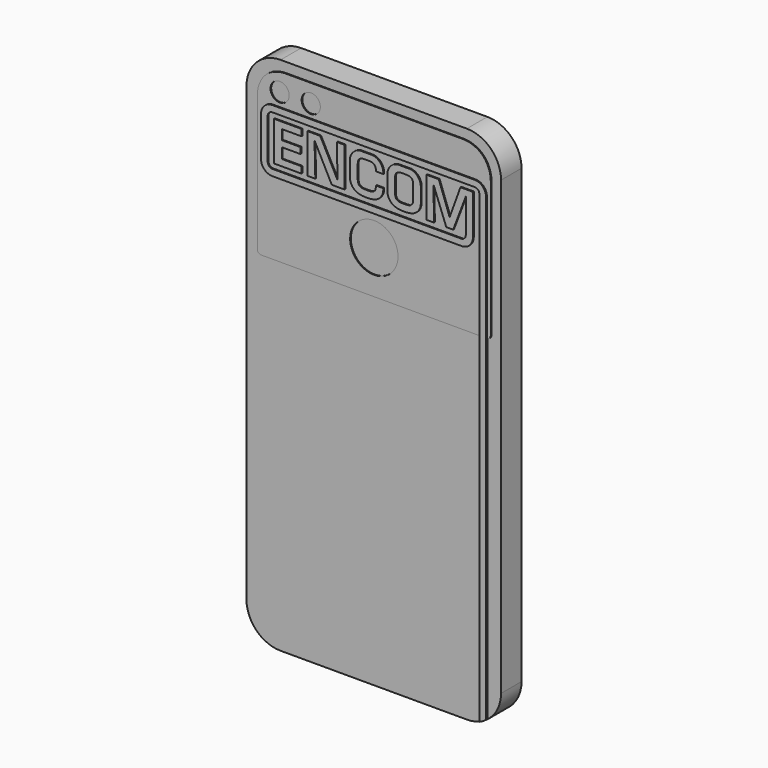
from build123d import *

# Parameters (mm, degrees)
F0_W     = 33.5805061566
F0_H     = 21.1181491613
F0_R     = 2.7798200703
F1_DEPTH = 7.62
F2_DEPTH = 0.254
F3_W     = 56.1288154928
F3_H     = 1.9038211044
F3_W_2   = 1.9916594028
F3_H_2   = 12.0399824588
F3_W_3   = 60.1634240953
F3_H_3   = 1.8881708384
F3_W_4   = 1.9932091236
F3_H_4   = 21.9200883571
F4_DEPTH = 0.5588


with BuildPart() as f1:
    # F0 (on Front) → F1 (new body)
    with BuildSketch(Plane.XZ):
        with BuildLine():
            Line((229.2512688186, 129.6003680688), (201.261898373, 129.6003680688))
            ThreePointArc((201.261898373, 129.6003680688), (194.0776934762, 126.6245729657), (191.101898373, 119.4403680688))
            Line((191.101898373, 119.4403680688), (191.101898373, -14.9256319312))
            ThreePointArc((191.101898373, -14.9256319312), (194.0776934762, -22.109836828), (201.261898373, -25.0856319312))
            Line((201.261898373, -25.0856319312), (229.2512688186, -25.0856319312))
            Line((229.2512688186, -25.0856319312), (229.2512688186, 76.8102183938))
            Line((229.2512688186, 76.8102183938), (195.670762662, 76.8102183938))
            ThreePointArc((195.670762662, 76.8102183938), (194.8754453058, 77.1396496291), (194.5460140705, 77.9349669853))
            Line((194.5460140705, 77.9349669853), (194.5460140705, 118.3175742626))
            ThreePointArc((194.5460140705, 118.3175742626), (194.9559900402, 120.9651454276), (196.1475163698, 123.3647242188))
            ThreePointArc((196.1475163698, 123.3647242188), (197.3925900387, 124.7286537572), (198.9371180534, 125.7410496473))
            ThreePointArc((198.9371180534, 125.7410496473), (200.6644568507, 126.3825901352), (202.4843841791, 126.6709268093))
            Line((202.4843841791, 126.6709268093), (229.2512688186, 126.6709268093))
            Line((229.2512688186, 126.6709268093), (229.2512688186, 129.6003680688))
        make_face()
        with BuildLine():
            Line((256.633898373, 129.6003680688), (229.2512688186, 129.6003680688))
            Line((229.2512688186, 129.6003680688), (229.2512688186, 126.6709268093))
            Line((229.2512688186, 126.6709268093), (256.018153458, 126.6709268093))
            ThreePointArc((256.018153458, 126.6709268093), (257.8380807864, 126.3825901352), (259.5654195837, 125.7410496473))
            ThreePointArc((259.5654195837, 125.7410496473), (261.1099475984, 124.7286537572), (262.3550212673, 123.3647242188))
            ThreePointArc((262.3550212673, 123.3647242188), (263.546547597, 120.9651454276), (263.9565235666, 118.3175742626))
            Line((263.9565235666, 118.3175742626), (263.9565235666, 77.9349669853))
            ThreePointArc((263.9565235666, 77.9349669853), (263.6270923313, 77.1396496291), (262.8317749751, 76.8102183938))
            Line((262.8317749751, 76.8102183938), (229.2512688186, 76.8102183938))
            Line((229.2512688186, 76.8102183938), (229.2512688186, -25.0856319312))
            Line((229.2512688186, -25.0856319312), (256.633898373, -25.0856319312))
            ThreePointArc((256.633898373, -25.0856319312), (263.8181032699, -22.109836828), (266.793898373, -14.9256319312))
            Line((266.793898373, -14.9256319312), (266.793898373, 119.4403680688))
            ThreePointArc((266.793898373, 119.4403680688), (263.8181032699, 126.6245729657), (256.633898373, 129.6003680688))
        make_face()
        with Locations((212.4610157403, 107.7584996819)):
            Rectangle(F0_W, F0_H)
        with Locations((246.0415218969, 107.7584996819)):
            Rectangle(F0_W, F0_H)
        with BuildLine():
            Line((262.8317749751, 97.1994251013), (229.2512688186, 97.1994251013))
            Line((229.2512688186, 97.1994251013), (229.2512688186, 96.7630286436))
            ThreePointArc((229.2512688186, 96.7630286436), (234.2846818006, 94.6781207214), (236.3695897228, 89.6447077394))
            ThreePointArc((236.3695897228, 89.6447077394), (234.2846818006, 84.6112947573), (229.2512688186, 82.5263868351))
            Line((229.2512688186, 82.5263868351), (229.2512688186, 77.9349669853))
            Line((229.2512688186, 77.9349669853), (262.8317749751, 77.9349669853))
            Line((262.8317749751, 77.9349669853), (262.8317749751, 97.1994251013))
        make_face()
        with BuildLine():
            Line((229.2512688186, 96.7630286436), (229.2512688186, 97.1994251013))
            Line((229.2512688186, 97.1994251013), (195.670762662, 97.1994251013))
            Line((195.670762662, 97.1994251013), (195.670762662, 77.9349669853))
            Line((195.670762662, 77.9349669853), (229.2512688186, 77.9349669853))
            Line((229.2512688186, 77.9349669853), (229.2512688186, 82.5263868351))
            ThreePointArc((229.2512688186, 82.5263868351), (222.1329479143, 89.6447077394), (229.2512688186, 96.7630286436))
        make_face()
        with BuildLine():
            Line((229.2512688186, 118.3175742626), (229.2512688186, 126.6709268093))
            Line((229.2512688186, 126.6709268093), (202.4843841791, 126.6709268093))
            ThreePointArc((202.4843841791, 126.6709268093), (200.6644568507, 126.3825901352), (198.9371180534, 125.7410496473))
            ThreePointArc((198.9371180534, 125.7410496473), (197.3925900387, 124.7286537572), (196.1475163698, 123.3647242188))
            ThreePointArc((196.1475163698, 123.3647242188), (194.9559900402, 120.9651454276), (194.5460140705, 118.3175742626))
            Line((194.5460140705, 118.3175742626), (194.5460140705, 77.9349669853))
            ThreePointArc((194.5460140705, 77.9349669853), (194.8754453058, 77.1396496291), (195.670762662, 76.8102183938))
            Line((195.670762662, 76.8102183938), (229.2512688186, 76.8102183938))
            Line((229.2512688186, 76.8102183938), (229.2512688186, 77.9349669853))
            Line((229.2512688186, 77.9349669853), (195.670762662, 77.9349669853))
            Line((195.670762662, 77.9349669853), (195.670762662, 97.1994251013))
            Line((195.670762662, 97.1994251013), (195.670762662, 118.3175742626))
            Line((195.670762662, 118.3175742626), (229.2512688186, 118.3175742626))
        make_face()
        with Locations((201.2345939875, 121.2812513113)):
            Circle(F0_R, mode=Mode.SUBTRACT)
        with Locations((210.4916423559, 121.2812513113)):
            Circle(F0_R, mode=Mode.SUBTRACT)
        with BuildLine():
            Line((256.018153458, 126.6709268093), (229.2512688186, 126.6709268093))
            Line((229.2512688186, 126.6709268093), (229.2512688186, 118.3175742626))
            Line((229.2512688186, 118.3175742626), (262.8317749751, 118.3175742626))
            Line((262.8317749751, 118.3175742626), (262.8317749751, 97.1994251013))
            Line((262.8317749751, 97.1994251013), (262.8317749751, 77.9349669853))
            Line((262.8317749751, 77.9349669853), (229.2512688186, 77.9349669853))
            Line((229.2512688186, 77.9349669853), (229.2512688186, 76.8102183938))
            Line((229.2512688186, 76.8102183938), (262.8317749751, 76.8102183938))
            ThreePointArc((262.8317749751, 76.8102183938), (263.6270923313, 77.1396496291), (263.9565235666, 77.9349669853))
            Line((263.9565235666, 77.9349669853), (263.9565235666, 118.3175742626))
            ThreePointArc((263.9565235666, 118.3175742626), (263.546547597, 120.9651454276), (262.3550212673, 123.3647242188))
            ThreePointArc((262.3550212673, 123.3647242188), (261.1099475984, 124.7286537572), (259.5654195837, 125.7410496473))
            ThreePointArc((259.5654195837, 125.7410496473), (257.8380807864, 126.3825901352), (256.018153458, 126.6709268093))
        make_face()
        with BuildLine():
            ThreePointArc((236.3695897228, 89.6447077394), (234.2846818006, 94.6781207214), (229.2512688186, 96.7630286436))
            Line((229.2512688186, 96.7630286436), (229.2512688186, 82.5263868351))
            ThreePointArc((229.2512688186, 82.5263868351), (234.2846818006, 84.6112947573), (236.3695897228, 89.6447077394))
        make_face()
        with BuildLine():
            Line((229.2512688186, 82.5263868351), (229.2512688186, 96.7630286436))
            ThreePointArc((229.2512688186, 96.7630286436), (222.1329479143, 89.6447077394), (229.2512688186, 82.5263868351))
        make_face()
        with Locations((210.4916423559, 121.2812513113)):
            Circle(F0_R)
        with Locations((201.2345939875, 121.2812513113)):
            Circle(F0_R)
    extrude(amount=-F1_DEPTH)


with BuildPart() as f2:
    # F0 (on Front) → F2 (new body)
    with BuildSketch(Plane.XZ):
        with BuildLine():
            Line((256.018153458, 126.6709268093), (229.2512688186, 126.6709268093))
            Line((229.2512688186, 126.6709268093), (229.2512688186, 118.3175742626))
            Line((229.2512688186, 118.3175742626), (262.8317749751, 118.3175742626))
            Line((262.8317749751, 118.3175742626), (262.8317749751, 97.1994251013))
            Line((262.8317749751, 97.1994251013), (262.8317749751, 77.9349669853))
            Line((262.8317749751, 77.9349669853), (229.2512688186, 77.9349669853))
            Line((229.2512688186, 77.9349669853), (229.2512688186, 76.8102183938))
            Line((229.2512688186, 76.8102183938), (262.8317749751, 76.8102183938))
            ThreePointArc((262.8317749751, 76.8102183938), (263.6270923313, 77.1396496291), (263.9565235666, 77.9349669853))
            Line((263.9565235666, 77.9349669853), (263.9565235666, 118.3175742626))
            ThreePointArc((263.9565235666, 118.3175742626), (263.546547597, 120.9651454276), (262.3550212673, 123.3647242188))
            ThreePointArc((262.3550212673, 123.3647242188), (261.1099475984, 124.7286537572), (259.5654195837, 125.7410496473))
            ThreePointArc((259.5654195837, 125.7410496473), (257.8380807864, 126.3825901352), (256.018153458, 126.6709268093))
        make_face()
        with BuildLine():
            Line((229.2512688186, 118.3175742626), (229.2512688186, 126.6709268093))
            Line((229.2512688186, 126.6709268093), (202.4843841791, 126.6709268093))
            ThreePointArc((202.4843841791, 126.6709268093), (200.6644568507, 126.3825901352), (198.9371180534, 125.7410496473))
            ThreePointArc((198.9371180534, 125.7410496473), (197.3925900387, 124.7286537572), (196.1475163698, 123.3647242188))
            ThreePointArc((196.1475163698, 123.3647242188), (194.9559900402, 120.9651454276), (194.5460140705, 118.3175742626))
            Line((194.5460140705, 118.3175742626), (194.5460140705, 77.9349669853))
            ThreePointArc((194.5460140705, 77.9349669853), (194.8754453058, 77.1396496291), (195.670762662, 76.8102183938))
            Line((195.670762662, 76.8102183938), (229.2512688186, 76.8102183938))
            Line((229.2512688186, 76.8102183938), (229.2512688186, 77.9349669853))
            Line((229.2512688186, 77.9349669853), (195.670762662, 77.9349669853))
            Line((195.670762662, 77.9349669853), (195.670762662, 97.1994251013))
            Line((195.670762662, 97.1994251013), (195.670762662, 118.3175742626))
            Line((195.670762662, 118.3175742626), (229.2512688186, 118.3175742626))
        make_face()
        with Locations((201.2345939875, 121.2812513113)):
            Circle(F0_R, mode=Mode.SUBTRACT)
        with Locations((210.4916423559, 121.2812513113)):
            Circle(F0_R, mode=Mode.SUBTRACT)
        with Locations((212.4610157403, 107.7584996819)):
            Rectangle(F0_W, F0_H)
        with BuildLine():
            Line((229.2512688186, 96.7630286436), (229.2512688186, 97.1994251013))
            Line((229.2512688186, 97.1994251013), (195.670762662, 97.1994251013))
            Line((195.670762662, 97.1994251013), (195.670762662, 77.9349669853))
            Line((195.670762662, 77.9349669853), (229.2512688186, 77.9349669853))
            Line((229.2512688186, 77.9349669853), (229.2512688186, 82.5263868351))
            ThreePointArc((229.2512688186, 82.5263868351), (222.1329479143, 89.6447077394), (229.2512688186, 96.7630286436))
        make_face()
        with BuildLine():
            Line((262.8317749751, 97.1994251013), (229.2512688186, 97.1994251013))
            Line((229.2512688186, 97.1994251013), (229.2512688186, 96.7630286436))
            ThreePointArc((229.2512688186, 96.7630286436), (234.2846818006, 94.6781207214), (236.3695897228, 89.6447077394))
            ThreePointArc((236.3695897228, 89.6447077394), (234.2846818006, 84.6112947573), (229.2512688186, 82.5263868351))
            Line((229.2512688186, 82.5263868351), (229.2512688186, 77.9349669853))
            Line((229.2512688186, 77.9349669853), (262.8317749751, 77.9349669853))
            Line((262.8317749751, 77.9349669853), (262.8317749751, 97.1994251013))
        make_face()
        with Locations((246.0415218969, 107.7584996819)):
            Rectangle(F0_W, F0_H)
    extrude(amount=F2_DEPTH)

    # F3 (on Front) → F4 (join)
    with BuildSketch(Plane.XZ):
        Polygon((199.7636705637, 102.2084653378), (207.9194486141, 102.2084653378), (207.9194486141, 104.1282191873), (202.0396590233, 104.1282191873), (202.0396590233, 107.2249636054), (207.5955271721, 107.2249636054), (207.5955271721, 108.1428825855), (207.5955271721, 109.0608015656), (202.0404785872, 109.0608015656), (202.0404785872, 111.972540617), (207.9194486141, 111.972540617), (207.9194486141, 113.9081418514), (199.7636705637, 113.9081418514), align=None)
        Polygon((218.5415214992, 108.1428825855), (220.7203507423, 108.1428825855), (220.7203507423, 113.9081418514), (218.4271961451, 113.9081418514), align=None)
        Polygon((216.9222682714, 102.2084653378), (220.7203507423, 102.2084653378), (220.7203507423, 108.1428825855), (218.5415214992, 108.1428825855), (218.6210900545, 104.1303575039), (218.5589185962, 104.129124641), (216.466729666, 108.1428825855), (213.8594988403, 108.1428825855), align=None)
        Polygon((211.8716859322, 111.9944657598), (213.8594988403, 108.1428825855), (216.466729666, 108.1428825855), (213.4615629911, 113.9081418514), (209.6930146217, 113.9081418514), (209.6930146217, 108.1428825855), (211.8812335809, 108.1428825855), (211.7895185947, 111.992508173), align=None)
        Polygon((209.6930146217, 102.2084653378), (212.0226174593, 102.2084653378), (211.8812335809, 108.1428825855), (209.6930146217, 108.1428825855), align=None)
        with BuildLine():
            Line((237.8193736076, 112.0741516352), (238.4150922298, 112.0741516352))
            Line((238.4150922298, 112.0741516352), (238.4150922298, 113.9081418514))
            Line((238.4150922298, 113.9081418514), (236.5544438362, 113.9081418514))
            ThreePointArc((236.5544438362, 113.9081418514), (236.3760720746, 113.8790212582), (236.1993858825, 113.8409885906))
            ThreePointArc((236.1993858825, 113.8409885906), (234.406717709, 112.7914019816), (233.4919741893, 110.9263187333))
            ThreePointArc((233.4919741893, 110.9263187333), (233.4804676636, 110.8516665608), (233.4705293179, 110.7767894864))
            Line((233.4705293179, 110.7767894864), (233.4260046482, 110.2137640119))
            Line((233.4260046482, 110.2137640119), (233.4260046482, 108.1428825855))
            Line((233.4260046482, 108.1428825855), (235.7074469328, 108.1428825855))
            Line((235.7074469328, 108.1428825855), (235.7074469328, 110.119998455))
            ThreePointArc((235.7074469328, 110.119998455), (235.7176531546, 110.2203330886), (235.7326234029, 110.3200682244))
            ThreePointArc((235.7326234029, 110.3200682244), (235.7389398189, 110.3974798809), (235.748488876, 110.4745595618))
            ThreePointArc((235.748488876, 110.4745595618), (235.7565008871, 110.5798212659), (235.7712805637, 110.684347721))
            ThreePointArc((235.7712805637, 110.684347721), (235.7927284766, 110.8131717547), (235.8253023796, 110.9396414565))
            ThreePointArc((235.8253023796, 110.9396414565), (235.8453327429, 111.0025957281), (235.8681549799, 111.0645925123))
            ThreePointArc((235.8681549799, 111.0645925123), (235.8976925729, 111.1509776233), (235.9335179955, 111.2349502134))
            ThreePointArc((235.9335179955, 111.2349502134), (236.1113058429, 111.5308226696), (236.3807154714, 111.7466176673))
            ThreePointArc((236.3807154714, 111.7466176673), (236.5149337847, 111.82207606), (236.6574833462, 111.8802838529))
            ThreePointArc((236.6574833462, 111.8802838529), (236.7353133018, 111.91133184), (236.8147769734, 111.9379213941))
            ThreePointArc((236.8147769734, 111.9379213941), (237.0337352549, 112.0021574719), (237.2594984469, 112.035323476))
            ThreePointArc((237.2594984469, 112.035323476), (237.4351597426, 112.0580823334), (237.6121905096, 112.0639953609))
            ThreePointArc((237.6121905096, 112.0639953609), (237.7156576662, 112.0716110431), (237.8193736076, 112.0741516352))
        make_face()
        with BuildLine():
            Line((241.1227375269, 108.1428825855), (243.4041798115, 108.1428825855))
            Line((243.4041798115, 108.1428825855), (243.4041798115, 110.2137640119))
            Line((243.4041798115, 110.2137640119), (243.3596551418, 110.7767894864))
            ThreePointArc((243.3596551418, 110.7767894864), (243.3497167961, 110.8516665608), (243.3382102704, 110.9263187333))
            ThreePointArc((243.3382102704, 110.9263187333), (242.4234667507, 112.7914019816), (240.6307985772, 113.8409885906))
            ThreePointArc((240.6307985772, 113.8409885906), (240.4541123851, 113.8790212582), (240.2757406235, 113.9081418514))
            Line((240.2757406235, 113.9081418514), (238.4150922298, 113.9081418514))
            Line((238.4150922298, 113.9081418514), (238.4150922298, 112.0741516352))
            Line((238.4150922298, 112.0741516352), (239.0108108521, 112.0741516352))
            ThreePointArc((239.0108108521, 112.0741516352), (239.1145267935, 112.0716110431), (239.2179939501, 112.0639953609))
            ThreePointArc((239.2179939501, 112.0639953609), (239.3950247171, 112.0580823334), (239.5706860128, 112.035323476))
            ThreePointArc((239.5706860128, 112.035323476), (239.7964492048, 112.0021574719), (240.0154074862, 111.9379213941))
            ThreePointArc((240.0154074862, 111.9379213941), (240.0948711579, 111.91133184), (240.1727011135, 111.8802838529))
            ThreePointArc((240.1727011135, 111.8802838529), (240.315250675, 111.82207606), (240.4494689882, 111.7466176673))
            ThreePointArc((240.4494689882, 111.7466176673), (240.7188786168, 111.5308226696), (240.8966664642, 111.2349502134))
            ThreePointArc((240.8966664642, 111.2349502134), (240.9324918868, 111.1509776233), (240.9620294798, 111.0645925123))
            ThreePointArc((240.9620294798, 111.0645925123), (240.9848517168, 111.0025957281), (241.0048820801, 110.9396414565))
            ThreePointArc((241.0048820801, 110.9396414565), (241.0374559831, 110.8131717547), (241.058903896, 110.684347721))
            ThreePointArc((241.058903896, 110.684347721), (241.0736835726, 110.5798212659), (241.0816955837, 110.4745595618))
            ThreePointArc((241.0816955837, 110.4745595618), (241.0912446408, 110.3974798809), (241.0975610568, 110.3200682244))
            ThreePointArc((241.0975610568, 110.3200682244), (241.1125313051, 110.2203330886), (241.1227375269, 110.119998455))
            Line((241.1227375269, 110.119998455), (241.1227375269, 108.1428825855))
        make_face()
        with BuildLine():
            Line((238.4150922298, 104.2116135359), (238.4150922298, 102.2084653378))
            ThreePointArc((238.4150922298, 102.2084653378), (239.3492531993, 102.2508418573), (240.2757406235, 102.3776233196))
            ThreePointArc((240.2757406235, 102.3776233196), (240.4541123851, 102.4067439128), (240.6307985772, 102.4447765804))
            ThreePointArc((240.6307985772, 102.4447765804), (242.4234667507, 103.4943631894), (243.3382102704, 105.3594464377))
            ThreePointArc((243.3382102704, 105.3594464377), (243.3497167961, 105.4340986102), (243.3596551418, 105.5089756846))
            Line((243.3596551418, 105.5089756846), (243.4041798115, 106.0720011592))
            Line((243.4041798115, 106.0720011592), (243.4041798115, 108.1428825855))
            Line((243.4041798115, 108.1428825855), (241.1227375269, 108.1428825855))
            Line((241.1227375269, 108.1428825855), (241.1227375269, 106.165766716))
            ThreePointArc((241.1227375269, 106.165766716), (241.1125313051, 106.0654320825), (241.0975610568, 105.9656969467))
            ThreePointArc((241.0975610568, 105.9656969467), (241.0912446408, 105.8882852901), (241.0816955837, 105.8112056093))
            ThreePointArc((241.0816955837, 105.8112056093), (241.0736835726, 105.7059439052), (241.058903896, 105.60141745))
            ThreePointArc((241.058903896, 105.60141745), (241.0374559831, 105.4725934163), (241.0048820801, 105.3461237145))
            ThreePointArc((241.0048820801, 105.3461237145), (240.9848517168, 105.283169443), (240.9620294798, 105.2211726587))
            ThreePointArc((240.9620294798, 105.2211726587), (240.9324918868, 105.1347875478), (240.8966664642, 105.0508149576))
            ThreePointArc((240.8966664642, 105.0508149576), (240.7188786168, 104.7549425014), (240.4494689882, 104.5391475037))
            ThreePointArc((240.4494689882, 104.5391475037), (240.315250675, 104.4636891111), (240.1727011135, 104.4054813182))
            ThreePointArc((240.1727011135, 104.4054813182), (240.0948711579, 104.3744333311), (240.0154074862, 104.347843777))
            ThreePointArc((240.0154074862, 104.347843777), (239.7964492048, 104.2836076991), (239.5706860128, 104.250441695))
            ThreePointArc((239.5706860128, 104.250441695), (239.3950247171, 104.2276828377), (239.2179939501, 104.2217698101))
            ThreePointArc((239.2179939501, 104.2217698101), (239.1145267935, 104.214154128), (239.0108108521, 104.2116135359))
            Line((239.0108108521, 104.2116135359), (238.4150922298, 104.2116135359))
        make_face()
        with BuildLine():
            ThreePointArc((236.5544438362, 102.3776233196), (237.4809312604, 102.2508418573), (238.4150922298, 102.2084653378))
            Line((238.4150922298, 102.2084653378), (238.4150922298, 104.2116135359))
            Line((238.4150922298, 104.2116135359), (237.8193736076, 104.2116135359))
            ThreePointArc((237.8193736076, 104.2116135359), (237.7156576662, 104.214154128), (237.6121905096, 104.2217698101))
            ThreePointArc((237.6121905096, 104.2217698101), (237.4351597426, 104.2276828377), (237.2594984469, 104.250441695))
            ThreePointArc((237.2594984469, 104.250441695), (237.0337352549, 104.2836076991), (236.8147769734, 104.347843777))
            ThreePointArc((236.8147769734, 104.347843777), (236.7353133018, 104.3744333311), (236.6574833462, 104.4054813182))
            ThreePointArc((236.6574833462, 104.4054813182), (236.5149337847, 104.4636891111), (236.3807154714, 104.5391475037))
            ThreePointArc((236.3807154714, 104.5391475037), (236.1113058429, 104.7549425014), (235.9335179955, 105.0508149576))
            ThreePointArc((235.9335179955, 105.0508149576), (235.8976925729, 105.1347875478), (235.8681549799, 105.2211726587))
            ThreePointArc((235.8681549799, 105.2211726587), (235.8453327429, 105.283169443), (235.8253023796, 105.3461237145))
            ThreePointArc((235.8253023796, 105.3461237145), (235.7927284766, 105.4725934163), (235.7712805637, 105.60141745))
            ThreePointArc((235.7712805637, 105.60141745), (235.7565008871, 105.7059439052), (235.748488876, 105.8112056093))
            ThreePointArc((235.748488876, 105.8112056093), (235.7389398189, 105.8882852901), (235.7326234029, 105.9656969467))
            ThreePointArc((235.7326234029, 105.9656969467), (235.7176531546, 106.0654320825), (235.7074469328, 106.165766716))
            Line((235.7074469328, 106.165766716), (235.7074469328, 108.1428825855))
            Line((235.7074469328, 108.1428825855), (233.4260046482, 108.1428825855))
            Line((233.4260046482, 108.1428825855), (233.4260046482, 106.0720011592))
            Line((233.4260046482, 106.0720011592), (233.4705293179, 105.5089756846))
            ThreePointArc((233.4705293179, 105.5089756846), (233.4804676636, 105.4340986102), (233.4919741893, 105.3594464377))
            ThreePointArc((233.4919741893, 105.3594464377), (234.406717709, 103.4943631894), (236.1993858825, 102.4447765804))
            ThreePointArc((236.1993858825, 102.4447765804), (236.3760720746, 102.4067439128), (236.5544438362, 102.3776233196))
        make_face()
        with BuildLine():
            Line((227.3379266262, 113.9081418514), (227.3379266262, 112.0741516352))
            Line((227.3379266262, 112.0741516352), (227.3467183113, 112.0741516352))
            Line((227.3467183113, 112.0741516352), (227.9424369335, 112.0741516352))
            ThreePointArc((227.9424369335, 112.0741516352), (228.0461528749, 112.0716110431), (228.1496200316, 112.0639953609))
            ThreePointArc((228.1496200316, 112.0639953609), (228.3266507986, 112.0580823334), (228.5023120942, 112.035323476))
            ThreePointArc((228.5023120942, 112.035323476), (228.7280752863, 112.0021574719), (228.9470335677, 111.9379213941))
            ThreePointArc((228.9470335677, 111.9379213941), (229.0264972393, 111.91133184), (229.104327195, 111.8802838529))
            ThreePointArc((229.104327195, 111.8802838529), (229.2468767565, 111.82207606), (229.3810950697, 111.7466176673))
            ThreePointArc((229.3810950697, 111.7466176673), (229.6505046983, 111.5308226696), (229.8282925456, 111.2349502134))
            ThreePointArc((229.8282925456, 111.2349502134), (229.8641179682, 111.1509776233), (229.8936555612, 111.0645925123))
            ThreePointArc((229.8936555612, 111.0645925123), (229.9164777982, 111.0025957281), (229.9365081615, 110.9396414565))
            ThreePointArc((229.9365081615, 110.9396414565), (229.9690820646, 110.8131717547), (229.9905299775, 110.684347721))
            ThreePointArc((229.9905299775, 110.684347721), (230.0053096541, 110.5798212659), (230.0133216651, 110.4745595618))
            ThreePointArc((230.0133216651, 110.4745595618), (230.0228707222, 110.3974798809), (230.0291871382, 110.3200682244))
            ThreePointArc((230.0291871382, 110.3200682244), (230.0441573866, 110.2203330886), (230.0543636084, 110.119998455))
            Line((230.0543636084, 110.119998455), (230.0543636084, 109.9947020411))
            Line((230.0543636084, 109.9947020411), (232.2537600994, 109.9947020411))
            Line((232.2537600994, 109.9947020411), (232.2537600994, 110.2149261945))
            Line((232.2537600994, 110.2149261945), (232.2092354298, 110.777951669))
            ThreePointArc((232.2092354298, 110.777951669), (232.199297084, 110.8528287434), (232.1877905583, 110.9274809159))
            ThreePointArc((232.1877905583, 110.9274809159), (231.2730470386, 112.7925641643), (229.4803788651, 113.8421507732))
            ThreePointArc((229.4803788651, 113.8421507732), (229.3078455553, 113.8793954681), (229.1336945986, 113.9081418514))
            Line((229.1336945986, 113.9081418514), (227.3379266262, 113.9081418514))
        make_face()
        with BuildLine():
            Line((222.2755849361, 108.1440447681), (222.2755849361, 108.1428825855))
            Line((222.2755849361, 108.1428825855), (224.6214896441, 108.1428825855))
            Line((224.6214896441, 108.1428825855), (224.6214896441, 110.119998455))
            ThreePointArc((224.6214896441, 110.119998455), (224.6316958658, 110.2203330886), (224.6466661142, 110.3200682244))
            ThreePointArc((224.6466661142, 110.3200682244), (224.6529825302, 110.3974798809), (224.6625315873, 110.4745595618))
            ThreePointArc((224.6625315873, 110.4745595618), (224.6705435983, 110.5798212659), (224.6853232749, 110.684347721))
            ThreePointArc((224.6853232749, 110.684347721), (224.7067711878, 110.8131717547), (224.7393450909, 110.9396414565))
            ThreePointArc((224.7393450909, 110.9396414565), (224.7593754542, 111.0025957281), (224.7821976912, 111.0645925123))
            ThreePointArc((224.7821976912, 111.0645925123), (224.8117352842, 111.1509776233), (224.8475607068, 111.2349502134))
            ThreePointArc((224.8475607068, 111.2349502134), (225.0253485541, 111.5308226696), (225.2947581827, 111.7466176673))
            ThreePointArc((225.2947581827, 111.7466176673), (225.428976496, 111.82207606), (225.5715260574, 111.8802838529))
            ThreePointArc((225.5715260574, 111.8802838529), (225.6493560131, 111.91133184), (225.7288196847, 111.9379213941))
            ThreePointArc((225.7288196847, 111.9379213941), (225.9477779661, 112.0021574719), (226.1735411582, 112.035323476))
            ThreePointArc((226.1735411582, 112.035323476), (226.3492024538, 112.0580823334), (226.5262332209, 112.0639953609))
            ThreePointArc((226.5262332209, 112.0639953609), (226.6297003775, 112.0716110431), (226.7334163189, 112.0741516352))
            Line((226.7334163189, 112.0741516352), (227.3291349411, 112.0741516352))
            Line((227.3291349411, 112.0741516352), (227.3379266262, 112.0741516352))
            Line((227.3379266262, 112.0741516352), (227.3379266262, 113.9081418514))
            Line((227.3379266262, 113.9081418514), (225.3956504369, 113.9081418514))
            ThreePointArc((225.3956504369, 113.9081418514), (225.2214994802, 113.8793954681), (225.0489661704, 113.8421507732))
            ThreePointArc((225.0489661704, 113.8421507732), (223.2562979969, 112.7925641643), (222.3415544772, 110.9274809159))
            ThreePointArc((222.3415544772, 110.9274809159), (222.3300479516, 110.8528287434), (222.3201096058, 110.777951669))
            Line((222.3201096058, 110.777951669), (222.2755849361, 110.2149261945))
            Line((222.2755849361, 110.2149261945), (222.2755849361, 108.1440447681))
        make_face()
        with BuildLine():
            ThreePointArc((225.4040241241, 102.3787855022), (226.3669942845, 102.2487525493), (227.3379266262, 102.2098875714))
            Line((227.3379266262, 102.2098875714), (227.3379266262, 104.2116135359))
            Line((227.3379266262, 104.2116135359), (227.3291349411, 104.2116135359))
            Line((227.3291349411, 104.2116135359), (226.7334163189, 104.2116135359))
            ThreePointArc((226.7334163189, 104.2116135359), (226.6297003775, 104.214154128), (226.5262332209, 104.2217698101))
            ThreePointArc((226.5262332209, 104.2217698101), (226.3492024538, 104.2276828377), (226.1735411582, 104.250441695))
            ThreePointArc((226.1735411582, 104.250441695), (225.9477779661, 104.2836076991), (225.7288196847, 104.347843777))
            ThreePointArc((225.7288196847, 104.347843777), (225.6493560131, 104.3744333311), (225.5715260574, 104.4054813182))
            ThreePointArc((225.5715260574, 104.4054813182), (225.428976496, 104.4636891111), (225.2947581827, 104.5391475037))
            ThreePointArc((225.2947581827, 104.5391475037), (225.0253485541, 104.7549425014), (224.8475607068, 105.0508149576))
            ThreePointArc((224.8475607068, 105.0508149576), (224.8117352842, 105.1347875478), (224.7821976912, 105.2211726587))
            ThreePointArc((224.7821976912, 105.2211726587), (224.7593754542, 105.283169443), (224.7393450909, 105.3461237145))
            ThreePointArc((224.7393450909, 105.3461237145), (224.7067711878, 105.4725934163), (224.6853232749, 105.60141745))
            ThreePointArc((224.6853232749, 105.60141745), (224.6705435983, 105.7059439052), (224.6625315873, 105.8112056093))
            ThreePointArc((224.6625315873, 105.8112056093), (224.6529825302, 105.8882852901), (224.6466661142, 105.9656969467))
            ThreePointArc((224.6466661142, 105.9656969467), (224.6316958658, 106.0654320825), (224.6214896441, 106.165766716))
            Line((224.6214896441, 106.165766716), (224.6214896441, 108.1428825855))
            Line((224.6214896441, 108.1428825855), (222.2755849361, 108.1428825855))
            Line((222.2755849361, 108.1428825855), (222.2755849361, 106.0731633418))
            Line((222.2755849361, 106.0731633418), (222.3201096058, 105.5101378673))
            ThreePointArc((222.3201096058, 105.5101378673), (222.3300479516, 105.4352607928), (222.3415544772, 105.3606086204))
            ThreePointArc((222.3415544772, 105.3606086204), (223.2562979969, 103.495525372), (225.0489661704, 102.445938763))
            ThreePointArc((225.0489661704, 102.445938763), (225.2256523625, 102.4079060955), (225.4040241241, 102.3787855022))
        make_face()
        with BuildLine():
            Line((227.3379266262, 104.2116135359), (227.3379266262, 102.2098875714))
            ThreePointArc((227.3379266262, 102.2098875714), (228.2353044509, 102.2553850225), (229.1253209114, 102.3787855022))
            ThreePointArc((229.1253209114, 102.3787855022), (229.303692673, 102.4079060955), (229.4803788651, 102.445938763))
            ThreePointArc((229.4803788651, 102.445938763), (231.2730470386, 103.495525372), (232.1877905583, 105.3606086204))
            ThreePointArc((232.1877905583, 105.3606086204), (232.199297084, 105.4352607928), (232.2092354298, 105.5101378673))
            Line((232.2092354298, 105.5101378673), (232.2537600994, 106.0731633418))
            Line((232.2537600994, 106.0731633418), (232.2537600994, 106.2910631299))
            Line((232.2537600994, 106.2910631299), (230.0543636084, 106.2910631299))
            Line((230.0543636084, 106.2910631299), (230.0543636084, 106.165766716))
            ThreePointArc((230.0543636084, 106.165766716), (230.0441573866, 106.0654320825), (230.0291871382, 105.9656969467))
            ThreePointArc((230.0291871382, 105.9656969467), (230.0228707222, 105.8882852901), (230.0133216651, 105.8112056093))
            ThreePointArc((230.0133216651, 105.8112056093), (230.0053096541, 105.7059439052), (229.9905299775, 105.60141745))
            ThreePointArc((229.9905299775, 105.60141745), (229.9690820646, 105.4725934163), (229.9365081615, 105.3461237145))
            ThreePointArc((229.9365081615, 105.3461237145), (229.9164777982, 105.283169443), (229.8936555612, 105.2211726587))
            ThreePointArc((229.8936555612, 105.2211726587), (229.8641179682, 105.1347875478), (229.8282925456, 105.0508149576))
            ThreePointArc((229.8282925456, 105.0508149576), (229.6505046983, 104.7549425014), (229.3810950697, 104.5391475037))
            ThreePointArc((229.3810950697, 104.5391475037), (229.2468767565, 104.4636891111), (229.104327195, 104.4054813182))
            ThreePointArc((229.104327195, 104.4054813182), (229.0264972393, 104.3744333311), (228.9470335677, 104.347843777))
            ThreePointArc((228.9470335677, 104.347843777), (228.7280752863, 104.2836076991), (228.5023120942, 104.250441695))
            ThreePointArc((228.5023120942, 104.250441695), (228.3266507986, 104.2276828377), (228.1496200316, 104.2217698101))
            ThreePointArc((228.1496200316, 104.2217698101), (228.0461528749, 104.214154128), (227.9424369335, 104.2116135359))
            Line((227.9424369335, 104.2116135359), (227.3467183113, 104.2116135359))
            Line((227.3467183113, 104.2116135359), (227.3379266262, 104.2116135359))
        make_face()
        Polygon((256.7622959614, 102.2084653378), (256.7622959614, 102.0197641448), (258.8952766269, 102.0197641448), (258.902490139, 114.0043064952), (255.1763653755, 114.0043064952), (251.9906163216, 105.2259132266), (251.9319951534, 105.2259132266), (248.7232983112, 114.0043064952), (245.0365126133, 114.0043064952), (245.0365126133, 113.9081418514), (245.0365126133, 108.1428825855), (245.0365126133, 102.2084653378), (247.3303228617, 102.2084653378), (247.1502870321, 112.0081096888), (247.2019113399, 112.0090581135), (250.9705126286, 102.2084653378), (253.0142366886, 102.2084653378), (256.7622959614, 112.0972558856), align=None)
        with BuildLine():
            Line((255.3781572386, 100.635625422), (255.3781572386, 98.7318043176))
            Line((255.3781572386, 98.7318043176), (255.6793465587, 98.7318043176))
            ThreePointArc((255.6793465587, 98.7318043176), (257.9360745098, 99.7412338469), (258.8952766269, 102.0197641448))
            Line((258.8952766269, 102.0197641448), (256.7622959614, 102.0197641448))
            ThreePointArc((256.7622959614, 102.0197641448), (256.3568911156, 101.0410302678), (255.3781572386, 100.635625422))
        make_face()
        with Locations((227.3137494922, 99.6837148698)):
            Rectangle(F3_W, F3_H)
        with Locations((196.8693733215, 108.0397553742)):
            Rectangle(F3_W_2, F3_H_2)
        with BuildLine():
            Line((197.865203023, 102.0197641448), (195.8735436201, 102.0197641448))
            ThreePointArc((195.8735436201, 102.0197641448), (196.8952727919, 99.69181752), (199.2493417458, 98.7318043176))
            Line((199.2493417458, 98.7318043176), (199.2493417458, 100.635625422))
            ThreePointArc((199.2493417458, 100.635625422), (198.2706078688, 101.0410302678), (197.865203023, 102.0197641448))
        make_face()
        with BuildLine():
            Line((199.2493417458, 115.4438853264), (199.2493417458, 117.3320561647))
            ThreePointArc((199.2493417458, 117.3320561647), (196.8921665513, 116.3863437364), (195.8735436201, 114.0597466036))
            Line((195.8735436201, 114.0597466036), (197.865203023, 114.0597466036))
            ThreePointArc((197.865203023, 114.0597466036), (198.2706078688, 115.0384804806), (199.2493417458, 115.4438853264))
        make_face()
        with Locations((229.3310537934, 116.3879707456)):
            Rectangle(F3_W_3, F3_H_3)
        with BuildLine():
            ThreePointArc((262.7901136875, 114.0597466036), (261.7661640256, 116.381962715), (259.4127658411, 117.3320561647))
            Line((259.4127658411, 117.3320561647), (259.4127658411, 115.4438853264))
            ThreePointArc((259.4127658411, 115.4438853264), (260.3914997181, 115.0384804806), (260.7969045639, 114.0597466036))
            Line((260.7969045639, 114.0597466036), (262.7901136875, 114.0597466036))
        make_face()
        Polygon((262.7901136875, 100.6499901414), (262.7901136875, 114.0597466036), (260.7969045639, 114.0597466036), (260.7969045639, 100.635625422), (260.7969045639, 98.7318043176), (262.7901136875, 98.7318043176), align=None)
        with Locations((261.7935091257, 87.7717601391)):
            Rectangle(F3_W_4, F3_H_4)
        with BuildLine():
            Line((262.7901136875, -22.9254011065), (262.7901136875, 76.8117159605))
            Line((262.7901136875, 76.8117159605), (260.7969045639, 76.8117159605))
            Line((260.7969045639, 76.8117159605), (260.7969045639, -24.1171177477))
            ThreePointArc((260.7969045639, -24.1171177477), (261.8287889448, -23.5802667908), (262.7901136875, -22.9254011065))
        make_face()
    extrude(amount=F4_DEPTH)


solid = Compound([f1.part, f2.part])
